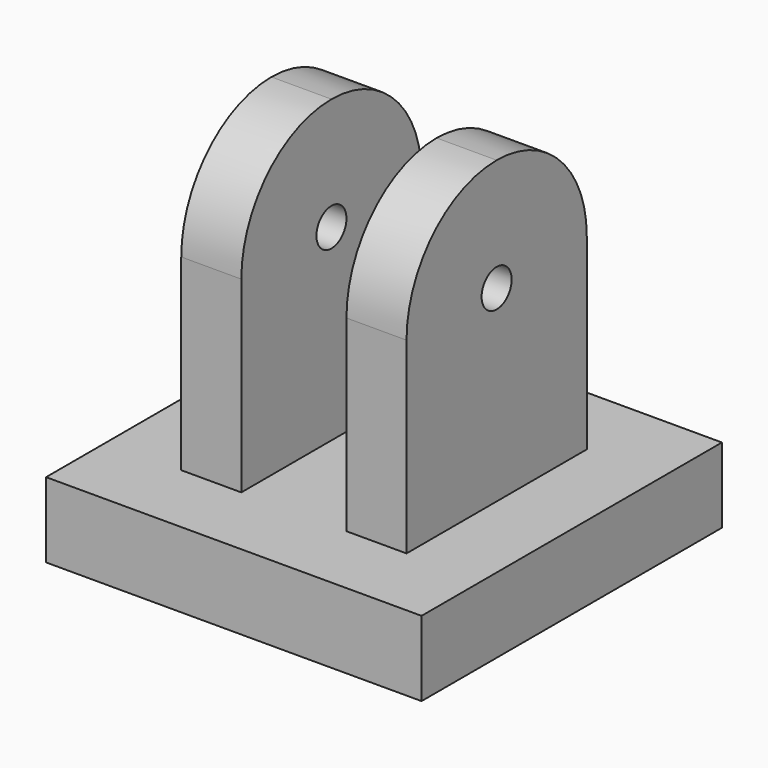
from build123d import *

# Parameters (mm, degrees)
F0_W     = 50
F0_H     = 50
F1_DEPTH = 10
F2_W     = 8
F2_H     = 30
F3_DEPTH = 40
F4_R     = 14.99999
F6_D     = 5


# Not quite as in the source:
# - a fillet or chamfer is up to 0.001 mm smaller than in the source, because OpenCascade refuses the exact size


with BuildPart() as f1:
    # F0 (on Top) → F1 (new body)
    with BuildSketch(Plane.XY):
        with Locations((1.0161269456, 0.1763854405)):
            Rectangle(F0_W, F0_H)
    extrude(amount=F1_DEPTH)

    # F2 (on face) → F3 (join)
    with BuildSketch(Plane.XY.offset(10)):
        with Locations((-9.9838730544, 0.1763854405)):
            Rectangle(F2_W, F2_H)
        with Locations((12.0161269456, 0.1763854405)):
            Rectangle(F2_W, F2_H)
    extrude(amount=F3_DEPTH)

    # F4 (radius 15 in the source; OpenCascade refuses exactly that, so slightly less here)
    f4_edges = [f1.edges().sort_by_distance(p)[0] for p in [
        (12.016127, -14.823615, 50),
        (12.016127, 15.176385, 50),
        (-9.983873, -14.823615, 50),
        (-9.983873, 15.176385, 50),
    ]]
    fillet(f4_edges, radius=F4_R)

    # F6 (through all)
    with Locations(Plane.YZ.offset(16.0161269456)):
        with Locations((0.1763854405, 35)):
            Hole(F6_D / 2)


solid = f1.part
